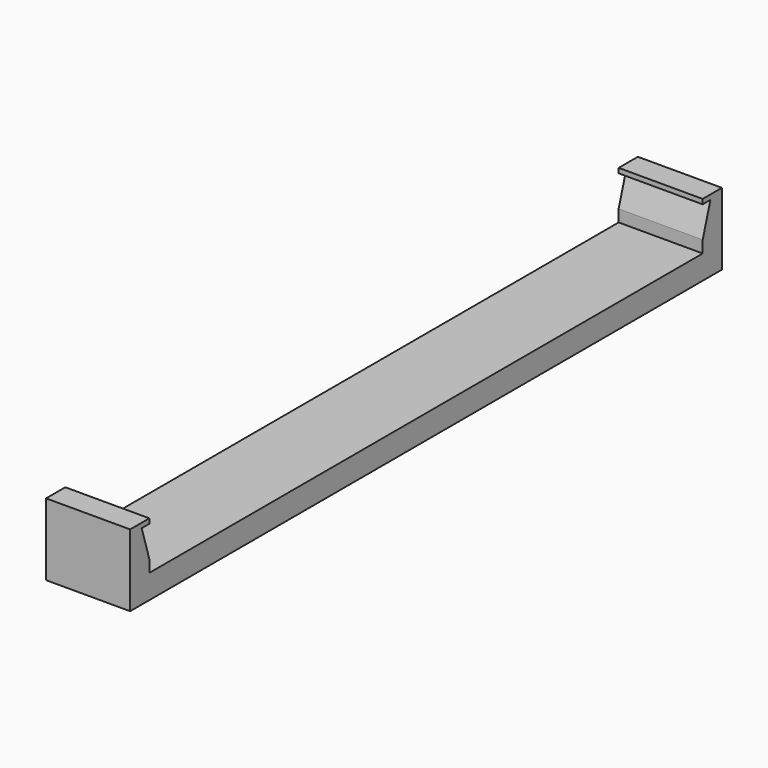
from build123d import *

# Parameters (mm, degrees)
F0_W     = 17.78
F0_H     = 73.152
F0_H_2   = 5.08
F1_DEPTH = 5.08
F2_DEPTH = 10.16
F4_DEPTH = 25.4


# Not quite as in the source:
# - a feature names something its author has since deleted; it is built from what else it names


with BuildPart() as f1:
    # F0 (on Top) → F1 (new body)
    with BuildSketch(Plane.XY):
        with Locations((8.89, -41.656)):
            Rectangle(F0_W, F0_H)
        with Locations((8.89, -2.54)):
            Rectangle(F0_W, F0_H_2)
        with Locations((8.89, -114.808)):
            Rectangle(F0_W, F0_H)
        with Locations((8.89, -153.924)):
            Rectangle(F0_W, F0_H_2)
    extrude(amount=-F1_DEPTH)

    # F0 (on Top) → F2 (join)
    with BuildSketch(Plane.XY):
        with Locations((8.89, -2.54)):
            Rectangle(F0_W, F0_H_2)
        with Locations((8.89, -153.924)):
            Rectangle(F0_W, F0_H_2)
    extrude(amount=F2_DEPTH)

    # F3 (on face) → F4 (cut)
    with BuildSketch(Plane(origin=(0, 0, 0), x_dir=(0, -1, 0), z_dir=(-1, 0, 0))):
        Polygon((3.048, 9.144), (5.08, 2.54), (5.08, 9.144), align=None)
        Polygon((151.384, 9.144), (151.384, 2.54), (153.416, 9.144), align=None)
    extrude(amount=-F4_DEPTH, mode=Mode.SUBTRACT)


solid = f1.part
